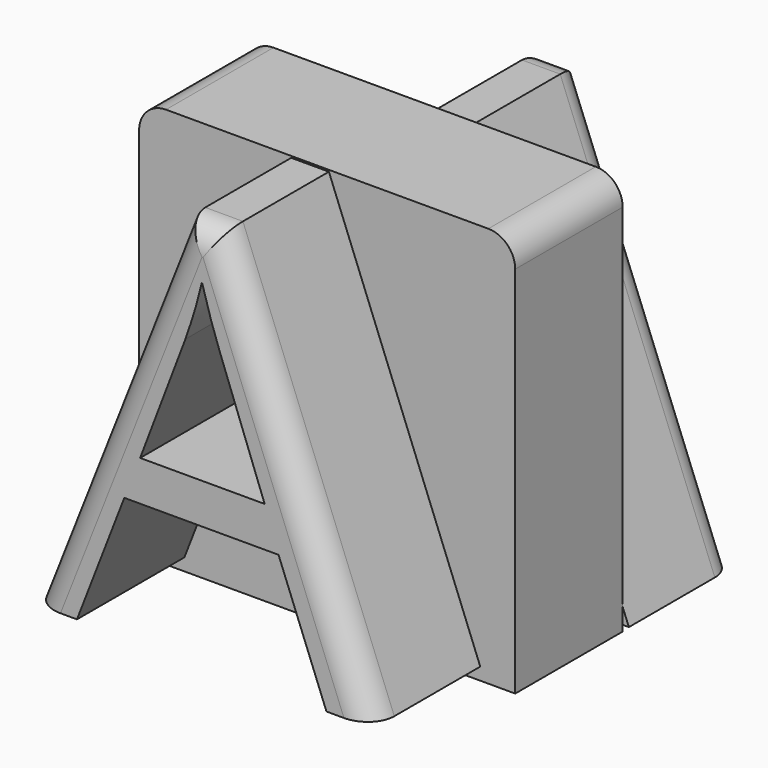
from build123d import *

# Parameters (mm, degrees)
F0_TEXT_SIZE = 100.3359462486
F1_DEPTH     = 25
F2_W         = 70
F2_H         = 74.5454568543
F3_DEPTH     = 25
F5_TEXT_SIZE = 101.9985979187
F6_DEPTH     = 25
F7_R         = 5
F8_R         = 5


# Not quite as in the source:
# - Text() gives the source's letters only with a copy of the font that has no kerning and outlines rounded to 1/6400 em; it was checked with that copy


with BuildPart() as f1:
    # F0 (on Front) → F1 (new body)
    with BuildSketch(Plane.XZ):
        with Locations((-70, -72.241881299)):
            Text('A', F0_TEXT_SIZE, font='Open Sans', text_align=(TextAlign.LEFT, TextAlign.BOTTOM))
    extrude(amount=F1_DEPTH)

    # F2 (on Front) + F1_face (on face) → F3 (join)
    with BuildSketch(Plane.XZ):
        with Locations((-35, -37.2727284272)):
            Rectangle(F2_W, F2_H)
    with BuildSketch(Plane(origin=(-38.1387729482, -25, -39.5044500859), x_dir=(1, 0, 0), z_dir=(0, -1, 0))):
        Polygon((14.0895008317, -9.9580359164), (23.0099935529, -32.7374312131), (31.6326139336, -32.7374312131), (3.460161526, 39.1909002538), (-3.5476772198, 39.1909002538), (-31.8612270518, -32.7374312131), (-23.4267365703, -32.7374312131), (-14.6159862903, -9.9580359164), align=None)
        with BuildLine():
            Line((3.1622891856, 19.7351331766), (11.5027147175, -2.4641949309))
            Line((11.5027147175, -2.4641949309), (-11.6686178693, -2.4641949309))
            Line((-11.6686178693, -2.4641949309), (-3.2498048794, 19.7351331766))
            add(Edge.make_bspline(
                [(-0.1613390339, 30.0666001419), (-1.2430859544, 25.3633526615), (-3.2498048794, 19.7351331766)],
                knots=[0, 0, 0, 1, 1, 1], degree=2))
            add(Edge.make_bspline(
                [(3.1622891856, 19.7351331766), (1.5475075507, 23.9523784173), (-0.1613390339, 30.0666001419)],
                knots=[0, 0, 0, 1, 1, 1], degree=2))
        make_face(mode=Mode.SUBTRACT)
    extrude(amount=F3_DEPTH)

    # F5 (on face) → F6 (join)
    with BuildSketch(Plane(origin=(0, 0, 0), x_dir=(-1, 0, 0), z_dir=(0, 1, 0))):
        with Locations((-1.1599593292, -73.4389905015)):
            Text('A', F5_TEXT_SIZE, font='Open Sans', text_align=(TextAlign.LEFT, TextAlign.BOTTOM))
    extrude(amount=F6_DEPTH)

    # F7
    f7_edges = [f1.edges().sort_by_distance(p)[0] for p in [
        (-70, -12.5, 0),
        (0, -12.5, 0),
    ]]
    fillet(f7_edges, radius=F7_R)

    # F8
    f8_edges = [f1.edges().sort_by_distance(p)[0] for p in [
        (-31.184752, 25, -0.318746),
        (-49.066382, 25, -36.878868),
        (-13.231405, 25, -36.878868),
        (-20.592385, -50, -36.277716),
        (-38.182531, -50, -0.31355),
        (-55.843225, -50, -36.277716),
    ]]
    fillet(f8_edges, radius=F8_R)


solid = f1.part
